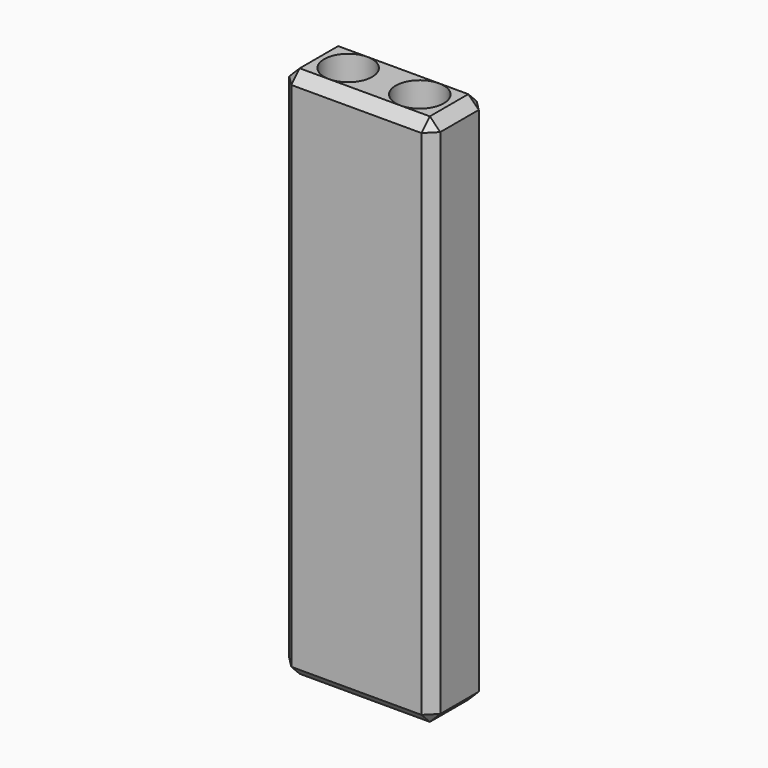
from build123d import *

# Parameters (mm, degrees)
F0_W     = 28.9
F0_H     = 13.2
F0_R     = 4.6
F1_DEPTH = 98
F2_DEPTH = 4
F3_SIZE  = 1.99999


# Not quite as in the source:
# - a fillet or chamfer is up to 0.001 mm smaller than in the source, because OpenCascade refuses the exact size


with BuildPart() as f1:
    # F0 (on Top) → F1 (new body)
    with BuildSketch(Plane.XY):
        with Locations((-11.3274157623, 0)):
            Rectangle(F0_W, F0_H)
        with Locations((-18.1774157623, 0)):
            Circle(F0_R, mode=Mode.SUBTRACT)
        with Locations((-4.4774157623, 0)):
            Circle(F0_R, mode=Mode.SUBTRACT)
    extrude(amount=F1_DEPTH)

    # F0 (on Top) → F2 (join)
    with BuildSketch(Plane.XY):
        with Locations((-11.3274157623, 0)):
            Rectangle(F0_W, F0_H)
        with Locations((-18.1774157623, 0)):
            Circle(F0_R, mode=Mode.SUBTRACT)
        with Locations((-4.4774157623, 0)):
            Circle(F0_R, mode=Mode.SUBTRACT)
        with Locations((-4.4774157623, 0)):
            Circle(F0_R)
        with Locations((-18.1774157623, 0)):
            Circle(F0_R)
    extrude(amount=-F2_DEPTH)

    # F3 (size 2 in the source; OpenCascade refuses exactly that, so slightly less here)
    f3_edges = [f1.edges().sort_by_distance(p)[0] for p in [
        (-11.327416, -6.6, 98),
        (3.122584, -6.6, 47),
        (-11.327416, -6.6, -4),
        (-25.777416, -6.6, 47),
        (-25.777416, 0, 98),
        (-25.777416, 0, -4),
        (-25.777416, 6.6, 47),
        (3.122584, 6.6, 47),
        (-11.327416, 6.6, 98),
        (-11.327416, 6.6, -4),
        (3.122584, 0, 98),
        (3.122584, 0, -4),
    ]]
    chamfer(f3_edges, length=F3_SIZE)


solid = f1.part
